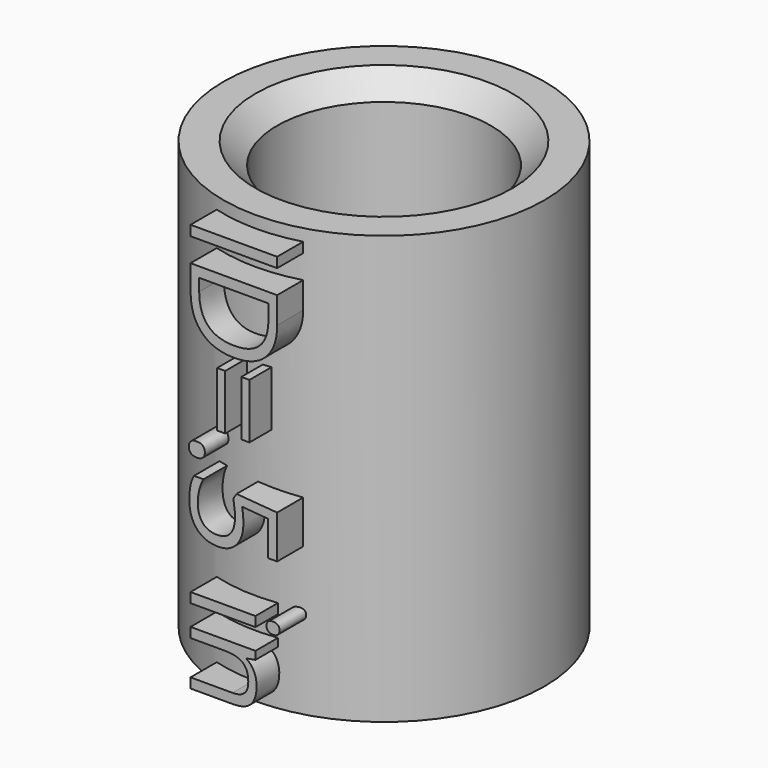
from build123d import *

# Parameters (mm, degrees)
F0_R         = 9.525
F0_R_2       = 6.35
F1_DEPTH     = 25.4
F3_TEXT_SIZE = 7.1989725876
F5_SIZE      = 1.27


# Not quite as in the source:
# - Text() gives the source's letters only with a copy of the font that has no kerning and outlines rounded to 1/6400 em; it was checked with that copy


with BuildPart() as f1:
    # F0 (on Top) → F1 (new body)
    with BuildSketch(Plane.XY):
        Circle(F0_R)
        Circle(F0_R_2, mode=Mode.SUBTRACT)
    extrude(amount=F1_DEPTH)

    # F3 (on offset) → F4 (join, up to the next surface of F1)
    with BuildSketch(Plane.XZ.offset(11.1125)):
        with Locations(Location((-2.5916301315, 25.4), (0, 0, -90))):
            Text('ID=.5 in', F3_TEXT_SIZE, font='Open Sans', text_align=(TextAlign.LEFT, TextAlign.BOTTOM))
    extrude(until=Until.NEXT, dir=(0, 1, 0))

    # F5
    f5_edges = [f1.edges().sort_by_distance(p)[0] for p in [
        (-6.35, 0, 25.4),
        (-6.35, 0, 0),
    ]]
    chamfer(f5_edges, length=F5_SIZE)


solid = f1.part
